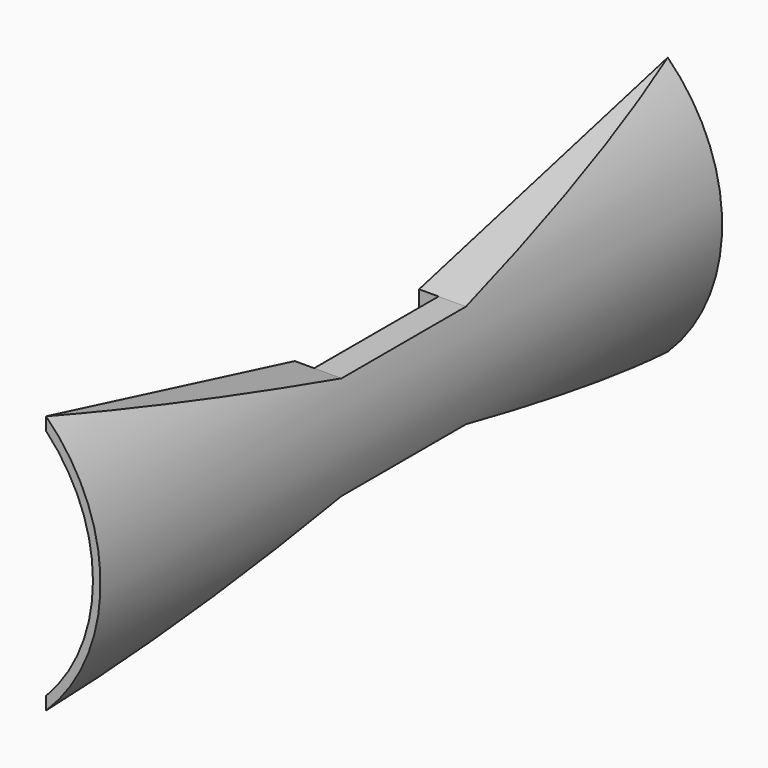
from build123d import *

# Parameters (mm, degrees)
F0_W      = 25
F0_H      = 100
F1_DEPTH  = 300
F3_DEPTH  = 80
F5_DEPTH  = 80
F7_DEPTH  = 15
F9_DEPTH  = 15
F11_DEPTH = 15
F13_DEPTH = 15
F15_DEPTH = 15
F17_DEPTH = 15
F19_DEPTH = 15
F21_DEPTH = 15
F23_DEPTH = 300
F24_W     = 7.5
F24_H     = 60
F25_DEPTH = 10
F26_W     = 2.5
F26_H     = 15
F27_DEPTH = 20
F28_W     = 10
F28_H     = 15
F29_DEPTH = 2.5


# Not quite as in the source:
# - a pattern or mirror of a feature is missing from the dataset's text; its kind, count and spacing are read off the source's solid


with BuildPart() as f1:
    # F0 (on Front) → F1 (new body)
    with BuildSketch(Plane.XZ):
        Rectangle(F0_W, F0_H)
    extrude(amount=F1_DEPTH)

    # F2 (on face) → F3 (cut)
    with BuildSketch(Plane.YZ.offset(12.5)):
        Polygon((-180, 20), (-120, 20), (0, 50), (-300, 50), align=None)
    extrude(amount=-F3_DEPTH, mode=Mode.SUBTRACT)

    # F4 (on face) → F5 (cut)
    with BuildSketch(Plane(origin=(-12.5, 0, 0), x_dir=(0, -1, 0), z_dir=(-1, 0, 0))):
        Polygon((180, -20), (120, -20), (0, -50), (300, -50), align=None)
    extrude(amount=-F5_DEPTH, mode=Mode.SUBTRACT)

    # F6 (on face) → F7 (cut)
    with BuildSketch(Plane.XZ.offset(300)):
        with BuildLine():
            Line((-12.5, 45), (-12.5, -45))
            ThreePointArc((-12.5, -45), (5.5958424018, 0), (-12.5, 45))
        make_face()
    f7 = extrude(amount=-F7_DEPTH, mode=Mode.SUBTRACT)

    # F7_copies: F7 across plane
    add(f7.mirror(Plane.ZX.offset(-150)), mode=Mode.SUBTRACT)

    # F8 (on face) → F9 (cut)
    with BuildSketch(Plane.XZ.offset(285)):
        with BuildLine():
            Line((-12.5, 40), (-12.5, -40))
            ThreePointArc((-12.5, -40), (2.77864045, 0), (-12.5, 40))
        make_face()
    f9 = extrude(amount=-F9_DEPTH, mode=Mode.SUBTRACT)

    # F9_copies: F9 across plane
    add(f9.mirror(Plane.ZX.offset(-150)), mode=Mode.SUBTRACT)

    # F10 (on face) → F11 (cut)
    with BuildSketch(Plane.XZ.offset(270)):
        with BuildLine():
            Line((-12.5, 35), (-12.5, -35))
            ThreePointArc((-12.5, -35), (-1.233971724, 0), (-12.5, 35))
        make_face()
    f11 = extrude(amount=-F11_DEPTH, mode=Mode.SUBTRACT)

    # F11_copies: F11 across plane
    add(f11.mirror(Plane.ZX.offset(-150)), mode=Mode.SUBTRACT)

    # F12 (on face) → F13 (cut)
    with BuildSketch(Plane.XZ.offset(255)):
        with BuildLine():
            Line((-12.5, 30), (-12.5, -30))
            ThreePointArc((-12.5, -30), (-4.4615242271, 0), (-12.5, 30))
        make_face()
    f13 = extrude(amount=-F13_DEPTH, mode=Mode.SUBTRACT)

    # F13_copies: F13 across plane
    add(f13.mirror(Plane.ZX.offset(-150)), mode=Mode.SUBTRACT)

    # F14 (on face) → F15 (cut)
    with BuildSketch(Plane.XZ.offset(240)):
        with BuildLine():
            Line((-12.5, 25), (-12.5, -25))
            ThreePointArc((-12.5, -25), (-7.0435605732, 0), (-12.5, 25))
        make_face()
    f15 = extrude(amount=-F15_DEPTH, mode=Mode.SUBTRACT)

    # F15_copies: F15 across plane
    add(f15.mirror(Plane.ZX.offset(-150)), mode=Mode.SUBTRACT)

    # F16 (on face) → F17 (cut)
    with BuildSketch(Plane.XZ.offset(225)):
        with BuildLine():
            Line((-12.5, 20), (-12.5, -20))
            ThreePointArc((-12.5, -20), (-9.0685424949, 0), (-12.5, 20))
        make_face()
    f17 = extrude(amount=-F17_DEPTH, mode=Mode.SUBTRACT)

    # F17_copies: F17 across plane
    add(f17.mirror(Plane.ZX.offset(-150)), mode=Mode.SUBTRACT)

    # F18 (on face) → F19 (cut)
    with BuildSketch(Plane.XZ.offset(210)):
        with BuildLine():
            Line((-12.5, 15), (-12.5, -15))
            ThreePointArc((-12.5, -15), (-10.5947501931, 0), (-12.5, 15))
        make_face()
    f19 = extrude(amount=-F19_DEPTH, mode=Mode.SUBTRACT)

    # F19_copies: F19 across plane
    add(f19.mirror(Plane.ZX.offset(-150)), mode=Mode.SUBTRACT)

    # F20 (on face) → F21 (cut)
    with BuildSketch(Plane.XZ.offset(195)):
        with BuildLine():
            Line((-12.5, 10), (-12.5, -10))
            ThreePointArc((-12.5, -10), (-11.660797831, 0), (-12.5, 10))
        make_face()
    f21 = extrude(amount=-F21_DEPTH, mode=Mode.SUBTRACT)

    # F21_copies: F21 across plane
    add(f21.mirror(Plane.ZX.offset(-150)), mode=Mode.SUBTRACT)

    # F22 (on face) → F23 (cut)
    with BuildSketch(Plane.XZ.offset(300)):
        with BuildLine():
            Line((12.5, 50), (-12.5, 50))
            ThreePointArc((-12.5, 50), (8.5102051443, 0), (-12.5, -50))
            Line((-12.5, -50), (12.5, -50))
            Line((12.5, -50), (12.5, 50))
        make_face()
    extrude(amount=-F23_DEPTH, mode=Mode.SUBTRACT)

    # F24 (on face) → F25 (cut)
    with BuildSketch(Plane.XY.offset(20)):
        with Locations((-8.75, -150)):
            Rectangle(F24_W, F24_H)
    extrude(amount=-F25_DEPTH, mode=Mode.SUBTRACT)

    # F26 (on face) → F27 (cut)
    with BuildSketch(Plane.XY.offset(10)):
        with Locations((-11.25, -162.5)):
            Rectangle(F26_W, F26_H)
        with Locations((-11.25, -137.5)):
            Rectangle(F26_W, F26_H)
    extrude(amount=-F27_DEPTH, mode=Mode.SUBTRACT)

    # F28 (on face) → F29 (cut)
    with BuildSketch(Plane(origin=(-12.5, 0, 0), x_dir=(0, -1, 0), z_dir=(-1, 0, 0))):
        with Locations((175, -2.5)):
            Rectangle(F28_W, F28_H)
    extrude(amount=-F29_DEPTH, mode=Mode.SUBTRACT)


solid = f1.part
